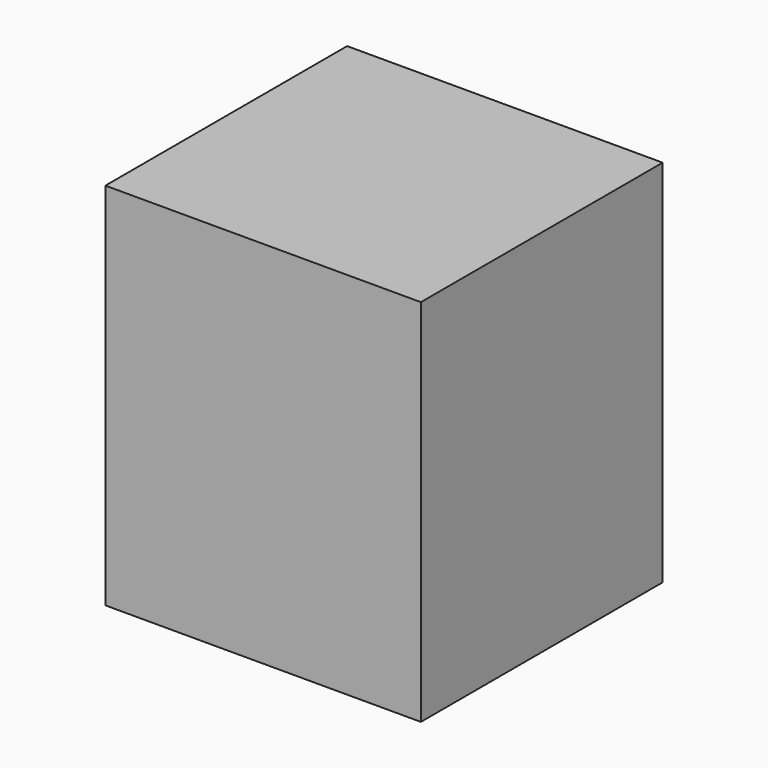
from build123d import *

# Parameters (mm, degrees)
F0_W     = 87.6123309135
F0_H     = 83.9102715254
F1_DEPTH = 102.616


# Not quite as in the source:
# - the program builds the solid bodies; features that only make, move or delete a surface that nothing else refers to are left out


with BuildPart() as f1:
    # F0 (on Top) → F1 (new body)
    with BuildSketch(Plane.XY):
        Rectangle(F0_W, F0_H)
    extrude(amount=F1_DEPTH)


solid = f1.part
